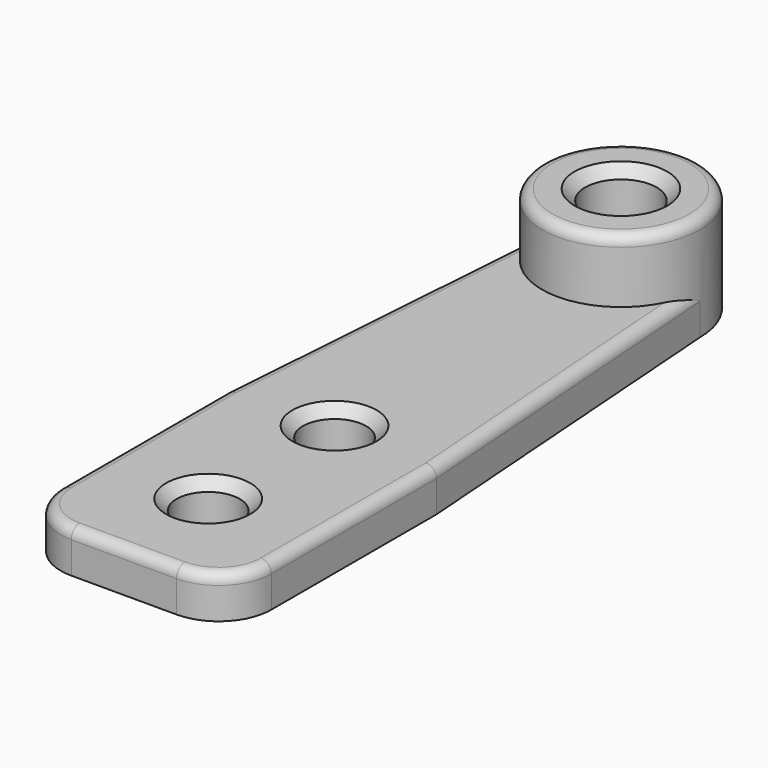
from build123d import *

# Parameters (mm, degrees)
F0_R         = 3
F1_DEPTH     = 4
F0_R_2       = 3.4
F2_DEPTH     = 10
F3_SIZE      = 1
F4_T1_DEPTH  = 22.1100533903
F4_T3_DEPTH  = 10
F4_T10_DEPTH = 44.4806964521
F4_S11_R     = 7.5
F4_T12_DEPTH = 24
F4_T14_ANGLE = 90
F4_T18_DEPTH = 44.4806964521
F4_S19_R     = 7.5
F4_T20_DEPTH = 24
F4_T22_ANGLE = 90


# Not quite as in the source:
# - a fillet or chamfer that OpenCascade refuses, or shapes differently, is made with other operations: its cross-section is extruded or revolved along the edge and cut away or added


with BuildPart() as f1:
    # F0 (on Top) → F1 (new body)
    with BuildSketch(Plane.XY):
        with BuildLine():
            Line((10, -34.3899466097), (7.5, 0))
            ThreePointArc((7.5, 0), (0, -7.5), (-7.5, 0))
            Line((-7.5, 0), (-10, -34.3899466097))
            Line((-10, -34.3899466097), (-10, -54))
            ThreePointArc((-10, -54), (-8.5355339059, -57.5355339059), (-5, -59))
            Line((-5, -59), (5, -59))
            ThreePointArc((5, -59), (8.5355339059, -57.5355339059), (10, -54))
            Line((10, -54), (10, -34.3899466097))
        make_face()
        with Locations((0, -49)):
            Circle(F0_R, mode=Mode.SUBTRACT)
        with Locations((0, -34)):
            Circle(F0_R, mode=Mode.SUBTRACT)
    extrude(amount=F1_DEPTH)

    # F0 (on Top) → F2 (join)
    with BuildSketch(Plane.XY):
        with BuildLine():
            ThreePointArc((-7.5, 0), (0, -7.5), (7.5, 0))
            ThreePointArc((7.5, 0), (0, 7.5), (-7.5, 0))
        make_face()
        Circle(F0_R_2, mode=Mode.SUBTRACT)
    extrude(amount=F2_DEPTH)

    # F3
    f3_edges = [f1.edges().sort_by_distance(p)[0] for p in [
        (-3, -34, 4),
        (-3, -49, 4),
        (-3.4, 0, 10),
    ]]
    chamfer(f3_edges, length=F3_SIZE)

    # F4: fillet of radius 1 on 5 edges, made by hand

    # F4_s2 → F4_t1 (cut)
    with BuildSketch(Plane.XZ.offset(31.8899466097)):
        with BuildLine():
            ThreePointArc((-9, 4), (-9.7071067812, 3.7071067812), (-10, 3))
            Line((-10, 3), (-10, 4))
            Line((-10, 4), (-9, 4))
        make_face()
        with BuildLine():
            ThreePointArc((9, 4), (9.7071067812, 3.7071067812), (10, 3))
            Line((10, 3), (10, 4))
            Line((10, 4), (9, 4))
        make_face()
    extrude(amount=F4_T1_DEPTH, mode=Mode.SUBTRACT)

    # F4_s4 → F4_t3 (cut)
    with BuildSketch(Plane.YZ.offset(-5)):
        with BuildLine():
            ThreePointArc((-58, 4), (-58.7071067812, 3.7071067812), (-59, 3))
            Line((-59, 3), (-59, 4))
            Line((-59, 4), (-58, 4))
        make_face()
    extrude(amount=F4_T3_DEPTH, mode=Mode.SUBTRACT)

    # F4_s5 → F4_t6 (revolve, cut)
    with BuildSketch(Plane.XZ):
        with BuildLine():
            ThreePointArc((7.5, 9), (7.2071067812, 9.7071067812), (6.5, 10))
            Line((6.5, 10), (7.5, 10))
            Line((7.5, 10), (7.5, 9))
        make_face()
    revolve(axis=Axis((0, 0, 10), (0, 0, -1)), mode=Mode.SUBTRACT)


with BuildPart() as f4_tool8:
    # F4_s9 → F4_t10 (new body)
    with BuildSketch(Plane(origin=(0.5043559293, 6.9379093918, 0), x_dir=(0, 0, 1), z_dir=(-0.072504336, -0.9973680972, 0))):
        with BuildLine():
            ThreePointArc((4, 6.4802607288), (3.7071067812, 7.18736751), (3, 7.4802607288))
            Line((3, 7.4802607288), (4, 7.4802607288))
            Line((4, 7.4802607288), (4, 6.4802607288))
        make_face()
    extrude(amount=F4_T10_DEPTH)

    # F4_s11 → F4_t12 (cut, symmetric)
    with BuildSketch(Plane.XY.offset(3.5)):
        Circle(F4_S11_R)
    extrude(amount=F4_T12_DEPTH, both=True, mode=Mode.SUBTRACT)


with BuildPart() as f1_1:
    add(f1.part)

    # F4_t7: cut F4_tool8
    add(f4_tool8.part, mode=Mode.SUBTRACT)

    # F4_s13 → F4_t14 (revolve, cut)
    with BuildSketch(Plane.XZ.offset(54)):
        with BuildLine():
            ThreePointArc((-9, 4), (-9.7071067812, 3.7071067812), (-10, 3))
            Line((-10, 3), (-10, 4))
            Line((-10, 4), (-9, 4))
        make_face()
    revolve(axis=Axis((-5, -54, 4), (0, 0, 1)), revolution_arc=F4_T14_ANGLE, mode=Mode.SUBTRACT)


with BuildPart() as f4_tool16:
    # F4_s17 → F4_t18 (new body)
    with BuildSketch(Plane(origin=(2.7206874304, -37.4257181897, 0), x_dir=(0, 0, 1), z_dir=(-0.072504336, 0.9973680972, 0))):
        with BuildLine():
            ThreePointArc((4, 6.4802607288), (3.7071067812, 7.18736751), (3, 7.4802607288))
            Line((3, 7.4802607288), (4, 7.4802607288))
            Line((4, 7.4802607288), (4, 6.4802607288))
        make_face()
    extrude(amount=F4_T18_DEPTH)

    # F4_s19 → F4_t20 (cut, symmetric)
    with BuildSketch(Plane.XY.offset(3.5)):
        Circle(F4_S19_R)
    extrude(amount=F4_T20_DEPTH, both=True, mode=Mode.SUBTRACT)


with BuildPart() as f1_2:
    add(f1_1.part)

    # F4_t15: cut F4_tool16
    add(f4_tool16.part, mode=Mode.SUBTRACT)

    # F4_s21 → F4_t22 (revolve, cut)
    with BuildSketch(Plane.YZ.offset(5)):
        with BuildLine():
            ThreePointArc((-58, 4), (-58.7071067812, 3.7071067812), (-59, 3))
            Line((-59, 3), (-59, 4))
            Line((-59, 4), (-58, 4))
        make_face()
    revolve(axis=Axis((5, -54, 4), (0, 0, 1)), revolution_arc=F4_T22_ANGLE, mode=Mode.SUBTRACT)


solid = f1_2.part
